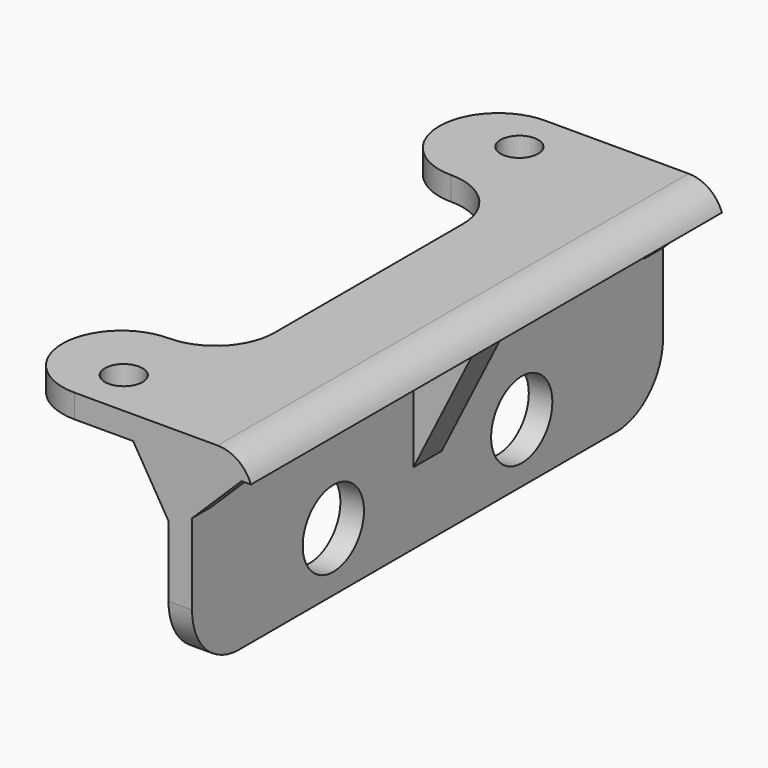
from build123d import *

# Parameters (mm, degrees)
F0_R        = 1.6
F1_DEPTH    = 2
F2_W        = 2
F2_H        = 50
F3_DEPTH    = 16
F4_R        = 1
F5_T1_DEPTH = 64.1421356237
F6_R        = 3.25
F7_DEPTH    = 25
F8_R        = 5
F10_DEPTH   = 1.5
F12_DEPTH   = 2
F14_DEPTH   = 2


# Not quite as in the source:
# - a fillet or chamfer that OpenCascade refuses, or shapes differently, is made with other operations: its cross-section is extruded or revolved along the edge and cut away or added
# - a feature names something its author has since deleted; it is built from what else it names


with BuildPart() as f1:
    # F0 (on Top) → F1 (new body)
    with BuildSketch(Plane.XY):
        with BuildLine():
            Line((10, 25), (-5, 25))
            ThreePointArc((-5, 25), (-8.5355339059, 23.5355339059), (-10, 20))
            ThreePointArc((-10, 20), (-8.5355339059, 16.4644660941), (-5, 15))
            ThreePointArc((-5, 15), (-1.4644660941, 13.5355339059), (0, 10))
            Line((0, 10), (0, -10))
            ThreePointArc((0, -10), (-1.4644660941, -13.5355339059), (-5, -15))
            ThreePointArc((-5, -15), (-8.5355339059, -16.4644660941), (-10, -20))
            ThreePointArc((-10, -20), (-8.5355339059, -23.5355339059), (-5, -25))
            Line((-5, -25), (10, -25))
            Line((10, -25), (10, 25))
        make_face()
        with Locations((-4, -21)):
            Circle(F0_R, mode=Mode.SUBTRACT)
        with Locations((-4, 21)):
            Circle(F0_R, mode=Mode.SUBTRACT)
    extrude(amount=F1_DEPTH)

    # F2 (on face) → F3 (join)
    with BuildSketch(Plane(origin=(0, 0, 0), x_dir=(1, 0, 0), z_dir=(0, 0, -1))):
        with Locations((4, 0)):
            Rectangle(F2_W, F2_H)
    extrude(amount=F3_DEPTH)

    # F4
    f4_edges = [f1.edges().sort_by_distance(p)[0] for p in [
        (3, 0, 0),
        (5, 0, 0),
    ]]
    fillet(f4_edges, radius=F4_R)

    # F5: fillet of radius 3 on 1 edges, made by hand

    # F5_s2 → F5_t1 (cut)
    with BuildSketch(Plane.XZ.offset(-32.0710678119)):
        with BuildLine():
            ThreePointArc((7.1715728753, 2), (8.9036236828, 1.4494897428), (10, 0))
            Line((10, 0), (10, 2))
            Line((10, 2), (7.1715728753, 2))
        make_face()
    extrude(amount=F5_T1_DEPTH, mode=Mode.SUBTRACT)

    # F6 (on face) → F7 (cut)
    with BuildSketch(Plane.YZ.offset(5)):
        with Locations((-10, -11)):
            Circle(F6_R)
        with Locations((10, -11)):
            Circle(F6_R)
    extrude(amount=-F7_DEPTH, mode=Mode.SUBTRACT)

    # F8
    f8_edges = [f1.edges().sort_by_distance(p)[0] for p in [
        (4, -25, -16),
        (4, 25, -16),
    ]]
    fillet(f8_edges, radius=F8_R)

    # F9 (on Front) → F10 (join, symmetric)
    with BuildSketch(Plane.XZ):
        Polygon((3.4634403419, 0), (0, 0), (3.4634403419, -10.6586683542), align=None)
        Polygon((4.6165082604, -10.6586683542), (9.9565815181, 0), (4.6165082604, 0), align=None)
    extrude(amount=F10_DEPTH, both=True)

    # F11 (on face) → F12 (join)
    with BuildSketch(Plane(origin=(0, 25, 0), x_dir=(-1, 0, 0), z_dir=(0, 1, 0))):
        with BuildLine():
            Line((-3, -5), (0, 0))
            Line((0, 0), (-2, 0))
            ThreePointArc((-2, 0), (-2.7071067812, -0.2928932188), (-3, -1))
            Line((-3, -1), (-3, -5))
        make_face()
        with BuildLine():
            Line((-9.370720014, 0), (-5, -4.2517034346))
            Line((-5, -4.2517034346), (-5, -1))
            ThreePointArc((-5, -1), (-5.2928932188, -0.2928932188), (-6, 0))
            Line((-6, 0), (-9.370720014, 0))
        make_face()
    extrude(amount=-F12_DEPTH)

    # F13 (on face) → F14 (join)
    with BuildSketch(Plane.XZ.offset(25)):
        with BuildLine():
            Line((0, 0), (3, -5))
            Line((3, -5), (3, -1))
            ThreePointArc((3, -1), (2.7071067812, -0.2928932188), (2, 0))
            Line((2, 0), (0, 0))
        make_face()
        with BuildLine():
            Line((5, -1), (5, -4.1425118317))
            Line((5, -4.1425118317), (9.2058293521, 0))
            Line((9.2058293521, 0), (6, 0))
            ThreePointArc((6, 0), (5.2928932188, -0.2928932188), (5, -1))
        make_face()
    extrude(amount=-F14_DEPTH)


solid = f1.part
